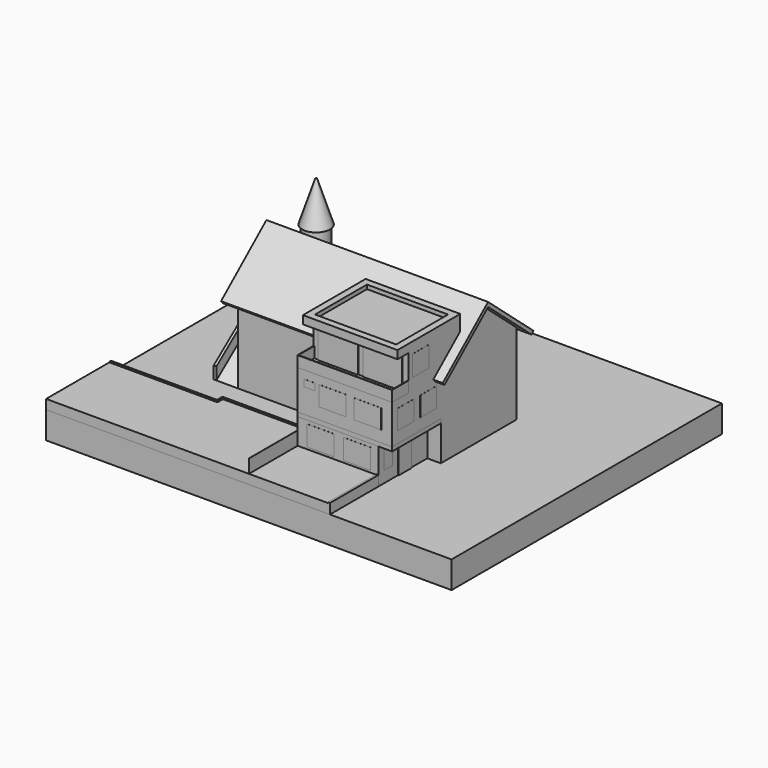
from build123d import *

# Parameters (mm, degrees)
F0_W      = 14000
F0_H      = 7000
F1_DEPTH  = 6000
F3_DEPTH  = 14000
F4_DEPTH  = 250
F5_DEPTH  = 250
F7_DEPTH  = 14000
F8_DEPTH  = 700
F9_DEPTH  = 700
F11_DEPTH = 700
F13_DEPTH = 700
F14_W     = 7000
F14_H     = 4500
F15_DEPTH = 9000
F16_DEPTH = 1800
F17_W     = 7000
F17_H     = 2600
F18_DEPTH = 1500
F19_DEPTH = 500
F20_W     = 6000
F20_H     = 4800
F21_DEPTH = 300
F22_W     = 7000
F22_H     = 300
F23_DEPTH = 4500
F24_DEPTH = 4500
F26_DEPTH = 800
F27_W     = 4500
F27_H     = 2600.45170784
F28_DEPTH = 1000
F29_W     = 1200
F29_H     = 2100
F30_DEPTH = 50
F31_W     = 6235.3289425373
F31_H     = 2381.1943054199
F32_DEPTH = 50
F33_W     = 400
F33_H     = 2600
F34_DEPTH = 500
F35_W     = 1500
F35_H     = 500
F36_DEPTH = 5
F37_W     = 2000
F37_H     = 1500
F38_DEPTH = 5
F39_W     = 1500
F39_H     = 500
F40_DEPTH = 5
F41_W     = 800
F41_H     = 1450.45170784
F42_DEPTH = 5
F43_W     = 800
F43_H     = 500
F44_DEPTH = 5
F43_W_2   = 2000
F43_H_2   = 1450
F43_H_3   = 1420.1555252075
F45_W     = 1500
F45_H     = 1450
F46_DEPTH = 5
F47_W     = 1500
F47_H     = 1530
F48_DEPTH = 5
F49_W     = 2200
F49_H     = 500
F50_DEPTH = 5
F51_W     = 30000
F51_H     = 25000
F52_DEPTH = 2000
F53_W     = 150
F53_H     = 0.9212493896
F53_H_2   = 4500
F54_DEPTH = 750
F53_W_2   = 7000
F53_H_3   = 150
F53_H_4   = 4500.9212493896
F55_DEPTH = 700
F56_W     = 10
F56_H     = 4500.9212493896
F57_DEPTH = 1000
F58_DEPTH = 1000
F59_DEPTH = 1000
F61_DEPTH = 1800
F63_DEPTH = 2000
F64_DEPTH = 50
F65_DEPTH = 50
F67_DEPTH = 2000
F68_DEPTH = 100
F69_DEPTH = 100
F71_DEPTH = 6000
F73_DEPTH = 200
F74_R     = 900
F75_DEPTH = 8500
F76_R     = 1050
F77_DEPTH = 3000


# Not quite as in the source:
# - a fillet or chamfer that OpenCascade refuses, or shapes differently, is made with other operations: its cross-section is extruded or revolved along the edge and cut away or added


with BuildPart() as f1:
    # F0 (on Top) → F1 (new body)
    with BuildSketch(Plane.XY):
        Rectangle(F0_W, F0_H)
    extrude(amount=F1_DEPTH)

    # F2 (on face) → F3 (join)
    with BuildSketch(Plane(origin=(-7000, 0, 0), x_dir=(0, -1, 0), z_dir=(-1, 0, 0))):
        Polygon((-3500, 6000), (0, 6000), (0, 8988.2593154907), align=None)
        Polygon((0, 8988.2593154907), (0, 6000), (3500, 6000), align=None)
    extrude(amount=-F3_DEPTH)

    # F4 (add, symmetric): a face of the model
    f4_faces = [f1.faces().sort_by_distance(p)[0] for p in [
        (0, 1750, 7494.1296577454),
    ]]
    extrude(f4_faces, amount=F4_DEPTH, both=True)

    # F5 (add, symmetric): a face of the model
    f5_faces = [f1.faces().sort_by_distance(p)[0] for p in [
        (0, -1750, 7494.1296577454),
    ]]
    extrude(f5_faces, amount=F5_DEPTH, both=True)

    # F6 (on face) → F7 (join)
    with BuildSketch(Plane(origin=(-7000, 0, 0), x_dir=(0, -1, 0), z_dir=(-1, 0, 0))):
        Polygon((0, 9316.9836101839), (-162.3298744643, 9178.3882503123), (0, 8988.2593154907), (162.3298744643, 9178.3882503123), align=None)
    extrude(amount=-F7_DEPTH)

    # F8 (add): a face of the model
    f8_faces = [f1.faces().sort_by_distance(p)[0] for p in [
        (0, 3581.1649372321, 6095.0644674108),
    ]]
    extrude(f8_faces, amount=F8_DEPTH)

    # F9 (add): a face of the model
    f9_faces = [f1.faces().sort_by_distance(p)[0] for p in [
        (0, -3581.1649372321, 6095.0644674108),
    ]]
    extrude(f9_faces, amount=F9_DEPTH)

    # F10 (on face) → F11 (join)
    with BuildSketch(Plane(origin=(-7000, 0, 0), x_dir=(0, -1, 0), z_dir=(-1, 0, 0))):
        Polygon((-4032.3610175005, 5545.4763515), (-3500, 6000), (0, 8917.555809021), (3500, 6000), (4032.3610175005, 5545.4763515), (4194.6908919648, 5735.6052863216), (0, 9316.9836101839), (-4194.6908919648, 5735.6052863216), align=None)
    extrude(amount=F11_DEPTH)

    # F12 (on face) → F13 (join)
    with BuildSketch(Plane.YZ.offset(7000)):
        Polygon((-4032.3610175005, 5545.4763515), (-3500, 6000), (0, 8988.2593154907), (3500, 6000), (4032.3610175005, 5545.4763515), (4194.6908919648, 5735.6052863216), (0, 9316.9836101839), (-4194.6908919648, 5735.6052863216), align=None)
    extrude(amount=F13_DEPTH)

    # F14 (on face) → F15 (join)
    with BuildSketch(Plane(origin=(0, 0, 0), x_dir=(1, 0, 0), z_dir=(0, 0, -1))):
        with Locations((3500, 5750)):
            Rectangle(F14_W, F14_H)
    extrude(amount=-F15_DEPTH)

    # F16 (add): a face of the model
    f16_faces = [f1.faces().sort_by_distance(p)[0] for p in [
        (3500, -3500, 7664.3621473466),
    ]]
    extrude(f16_faces, amount=F16_DEPTH)

    # F17 (on face) → F18 (cut)
    with BuildSketch(Plane.XZ.offset(8000)):
        with Locations((3500, 7100)):
            Rectangle(F17_W, F17_H)
    extrude(amount=-F18_DEPTH, mode=Mode.SUBTRACT)

    # F19 (cut): a face of the model
    f19_faces = [f1.faces().sort_by_distance(p)[0] for p in [
        (3500, -8000, 8700),
    ]]
    extrude(f19_faces, amount=-F19_DEPTH, mode=Mode.SUBTRACT)

    # F20 (on face) → F21 (cut)
    with BuildSketch(Plane.XY.offset(9000)):
        with Locations((3500, -4600)):
            Rectangle(F20_W, F20_H)
    extrude(amount=-F21_DEPTH, mode=Mode.SUBTRACT)


with BuildPart() as f23:
    # F22 (on face) → F23 (new body)
    with BuildSketch(Plane.XZ.offset(8000)):
        with Locations((3500, 2750)):
            Rectangle(F22_W, F22_H)
    extrude(amount=-F23_DEPTH)


with BuildPart() as f24:
    # F22 (on face) → F24 (new body)
    with BuildSketch(Plane.XZ.offset(8000)):
        with Locations((3500, 5650)):
            Rectangle(F22_W, F22_H)
    extrude(amount=-F24_DEPTH)


with BuildPart() as f26:
    # F25 (on face) → F26 (new body)
    with BuildSketch(Plane.XY.offset(5800)):
        Polygon((6960, -7960), (40, -7960), (40, -6500), (0, -6500), (0, -8000), (7000, -8000), (7000, -6500), (6960, -6500), align=None)
    extrude(amount=F26_DEPTH)


with BuildPart() as f28_tool:
    # F27 (on face) → F28 (new body)
    with BuildSketch(Plane.YZ.offset(7000)):
        with Locations((-5750, 1300.22585392)):
            Rectangle(F27_W, F27_H)
    extrude(amount=-F28_DEPTH)


with BuildPart() as f1_1:
    add(f1.part)

    # F28: cut by f28_tool
    add(f28_tool.part, mode=Mode.SUBTRACT)

    # F51 (on face) → F52 (join)
    with BuildSketch(Plane(origin=(0, 0, 0), x_dir=(1, 0, 0), z_dir=(0, 0, -1))):
        Rectangle(F51_W, F51_H)
    extrude(amount=F52_DEPTH)

    # F58 (add): a face of the model
    f58_faces = [f1_1.faces().sort_by_distance(p)[0] for p in [
        (-7000, 0, 3776.9399273598),
    ]]
    extrude(f58_faces, amount=F58_DEPTH)

    # F59 (add): a face of the model
    f59_faces = [f1_1.faces().sort_by_distance(p)[0] for p in [
        (-7700, 4043.5725637348, 5700.2662109964),
    ]]
    extrude(f59_faces, amount=F59_DEPTH)

    # F60 (on face) → F61 (join)
    with BuildSketch(Plane(origin=(-8000, 0, 0), x_dir=(0, -1, 0), z_dir=(-1, 0, 0))):
        Polygon((-2000, 0), (3500, 0), (1224.4793365597, 1777.8315871649), (1224.4793365597, 4500), (-2000, 4500), align=None)
    extrude(amount=F61_DEPTH)

    # F62 (on face) → F63 (join)
    with BuildSketch(Plane(origin=(-8000, 0, 0), x_dir=(0, -1, 0), z_dir=(-1, 0, 0))):
        Polygon((1224.4793365597, 4500), (-387.7603317201, 5825.6425857544), (-2000, 4500), align=None)
    extrude(amount=F63_DEPTH)

    # F64 (add): a face of the model
    f64_faces = [f1_1.faces().sort_by_distance(p)[0] for p in [
        (-9000, -418.3595024198, 5162.8212928772),
    ]]
    extrude(f64_faces, amount=F64_DEPTH)

    # F65 (add): a face of the model
    f65_faces = [f1_1.faces().sort_by_distance(p)[0] for p in [
        (-9000, 1193.8801658601, 5162.8212928772),
    ]]
    extrude(f65_faces, amount=F65_DEPTH)

    # F66 (on face) → F67 (join)
    with BuildSketch(Plane(origin=(-10000, 0, 0), x_dir=(0, -1, 0), z_dir=(-1, 0, 0))):
        Polygon((-387.7603317201, 5890.3742076897), (-419.5159347551, 5864.263586206), (-387.7603317201, 5825.6425857544), (-356.0047286852, 5864.263586206), align=None)
    extrude(amount=-F67_DEPTH)

    # F68 (add): a face of the model
    f68_faces = [f1_1.faces().sort_by_distance(p)[0] for p in [
        (-9000, 2015.8778015175, 4519.3105002258),
    ]]
    extrude(f68_faces, amount=F68_DEPTH)

    # F69 (add): a face of the model
    f69_faces = [f1_1.faces().sort_by_distance(p)[0] for p in [
        (-9000, -1240.3571380772, 4519.3105002258),
    ]]
    extrude(f69_faces, amount=F69_DEPTH)

    # F70 (on face) → F71 (cut)
    with BuildSketch(Plane.XZ.offset(3500)):
        Polygon((-10200, 4190.3742076897), (-8400, 5990.3742076897), (-10200, 5990.3742076897), align=None)
    extrude(amount=-F71_DEPTH, mode=Mode.SUBTRACT)

    # F72 (on face) → F73 (join)
    with BuildSketch(Plane(origin=(-9800, 0, 0), x_dir=(0, -1, 0), z_dir=(-1, 0, 0))):
        Polygon((1224.4793365597, 2685.697555542), (1224.4793365597, 1777.8315871649), (3500, 0), (3500, 907.8659683771), align=None)
    extrude(amount=-F73_DEPTH)

    # F74 (on face) → F75 (join)
    with BuildSketch(Plane.XY):
        with Locations((-7100, 2600)):
            Circle(F74_R)
    extrude(amount=F75_DEPTH)

    # F76 (on face) → F77 (join)
    with BuildSketch(Plane.XY.offset(8500)):
        with Locations((-7100, 2600)):
            Circle(F76_R)
    extrude(amount=F77_DEPTH)

    # F78: chamfer of 1000 x 3077.6835371753 on 1 edges, made by hand

    # F78_s1 → F78_t2 (revolve, cut)
    with BuildSketch(Plane.XZ.offset(-2600)):
        Polygon((-6050, 8422.3164628247), (-7050, 11500), (-6050, 11500), align=None)
    revolve(axis=Axis((-7100, 2600, 11500), (0, 0, 1)), mode=Mode.SUBTRACT)


with BuildPart() as f23_1:
    add(f23.part)

    # F28: cut by f28_tool
    add(f28_tool.part, mode=Mode.SUBTRACT)


with BuildPart() as f30:
    # F29 (on face) → F30 (new body, symmetric)
    with BuildSketch(Plane.YZ.offset(6000)):
        with Locations((-5600, 1050)):
            Rectangle(F29_W, F29_H)
    extrude(amount=F30_DEPTH, both=True)


with BuildPart() as f32:
    # F31 (on face) → F32 (new body, symmetric)
    with BuildSketch(Plane.XZ.offset(6500)):
        with Locations((3466.3508981466, 6990.59715271)):
            Rectangle(F31_W, F31_H)
    extrude(amount=F32_DEPTH, both=True)

    # F33 (on face) → F34 (cut)
    with BuildSketch(Plane.XZ.offset(6500)):
        with Locations((3500, 7100)):
            Rectangle(F33_W, F33_H)
    extrude(amount=F34_DEPTH, mode=Mode.SUBTRACT)


with BuildPart() as f36:
    # F35 (on face) → F36 (new body, symmetric)
    with BuildSketch(Plane(origin=(0, 0, 0), x_dir=(0, -1, 0), z_dir=(-1, 0, 0))):
        with Locations((6750, 2150)):
            Rectangle(F35_W, F35_H)
    extrude(amount=F36_DEPTH, both=True)


with BuildPart() as f36b:
    # F35 (on face) → F36, piece 2 (new body, symmetric)
    with BuildSketch(Plane(origin=(0, 0, 0), x_dir=(0, -1, 0), z_dir=(-1, 0, 0))):
        with Locations((4750, 2150)):
            Rectangle(F35_W, F35_H)
    extrude(amount=F36_DEPTH, both=True)


with BuildPart() as f38:
    # F37 (on face) → F38 (new body, symmetric)
    with BuildSketch(Plane.XZ.offset(8000)):
        with Locations((1700, 1600)):
            Rectangle(F37_W, F37_H)
    extrude(amount=F38_DEPTH, both=True)


with BuildPart() as f38b:
    # F37 (on face) → F38, piece 2 (new body, symmetric)
    with BuildSketch(Plane.XZ.offset(8000)):
        with Locations((4400, 1600)):
            Rectangle(F37_W, F37_H)
    extrude(amount=F38_DEPTH, both=True)


with BuildPart() as f40:
    # F39 (on face) → F40 (new body, symmetric)
    with BuildSketch(Plane(origin=(0, 0, 0), x_dir=(0, -1, 0), z_dir=(-1, 0, 0))):
        with Locations((4750, 4950)):
            Rectangle(F39_W, F39_H)
    extrude(amount=F40_DEPTH, both=True)


with BuildPart() as f40b:
    # F39 (on face) → F40, piece 2 (new body, symmetric)
    with BuildSketch(Plane(origin=(0, 0, 0), x_dir=(0, -1, 0), z_dir=(-1, 0, 0))):
        with Locations((6750, 4950)):
            Rectangle(F39_W, F39_H)
    extrude(amount=F40_DEPTH, both=True)


with BuildPart() as f42:
    # F41 (on face) → F42 (new body, symmetric)
    with BuildSketch(Plane.YZ.offset(6000)):
        with Locations((-7100, 1575.22585392)):
            Rectangle(F41_W, F41_H)
    extrude(amount=F42_DEPTH, both=True)


with BuildPart() as f44:
    # F43 (on face) → F44 (new body, symmetric)
    with BuildSketch(Plane.XZ.offset(8000)):
        with Locations((900, 4950)):
            Rectangle(F43_W, F43_H)
    extrude(amount=F44_DEPTH, both=True)


with BuildPart() as f44b:
    # F43 (on face) → F44, piece 2 (new body, symmetric)
    with BuildSketch(Plane.XZ.offset(8000)):
        with Locations((2600, 4475)):
            Rectangle(F43_W_2, F43_H_2)
    extrude(amount=F44_DEPTH, both=True)


with BuildPart() as f44c:
    # F43 (on face) → F44, piece 3 (new body, symmetric)
    with BuildSketch(Plane.XZ.offset(8000)):
        with Locations((5200, 4460.0777626038)):
            Rectangle(F43_W_2, F43_H_3)
    extrude(amount=F44_DEPTH, both=True)


with BuildPart() as f46:
    # F45 (on face) → F46 (new body, symmetric)
    with BuildSketch(Plane.YZ.offset(7000)):
        with Locations((-6750, 4475)):
            Rectangle(F45_W, F45_H)
    extrude(amount=F46_DEPTH, both=True)


with BuildPart() as f46b:
    # F45 (on face) → F46, piece 2 (new body, symmetric)
    with BuildSketch(Plane.YZ.offset(7000)):
        with Locations((-4650, 4475)):
            Rectangle(F45_W, F45_H)
    extrude(amount=F46_DEPTH, both=True)


with BuildPart() as f48:
    # F47 (on face) → F48 (new body, symmetric)
    with BuildSketch(Plane.YZ.offset(7000)):
        with Locations((-5350, 7415)):
            Rectangle(F47_W, F47_H)
    extrude(amount=F48_DEPTH, both=True)


with BuildPart() as f50:
    # F49 (on face) → F50 (new body, symmetric)
    with BuildSketch(Plane(origin=(0, 0, 0), x_dir=(0, -1, 0), z_dir=(-1, 0, 0))):
        with Locations((5000, 7931.1943054199)):
            Rectangle(F49_W, F49_H)
    extrude(amount=F50_DEPTH, both=True)


with BuildPart() as f54:
    # F53 (on face) → F54 (new body)
    with BuildSketch(Plane.XY):
        with Locations((5925, -7999.5393753052)):
            Rectangle(F53_W, F53_H)
        with Locations((5925, -10250)):
            Rectangle(F53_W, F53_H_2)
    extrude(amount=F54_DEPTH)


with BuildPart() as f54b:
    # F53 (on face) → F54, piece 2 (new body)
    with BuildSketch(Plane.XY):
        with Locations((-3500, -6075)):
            Rectangle(F53_W_2, F53_H_3)
        Polygon((-7000, -6150), (-7000, -6000), (-7150, -6000), (-7150, -6500), (-15000, -6500), (-15000, -6650), (-7000, -6650), align=None)
    extrude(amount=F54_DEPTH)


with BuildPart() as f55:
    # F53 (on face) → F55 (new body)
    with BuildSketch(Plane.XY):
        with Locations((-3500, -6075)):
            Rectangle(F53_W_2, F53_H_3)
        Polygon((-7000, -6150), (-7000, -6000), (-7150, -6000), (-7150, -6500), (-15000, -6500), (-15000, -6650), (-7000, -6650), align=None)
        Polygon((0, -7999.0787506104), (0, -6150), (-7000, -6150), (-7000, -6650), (-15000, -6650), (-15000, -12500), (5850, -12500), (5850, -7999.0787506104), align=None)
        with Locations((5925, -10249.5393753052)):
            Rectangle(F53_W, F53_H_4)
    extrude(amount=F55_DEPTH)


with BuildPart() as f57:
    # F56 (on face) → F57 (new body)
    with BuildSketch(Plane.XY.offset(700)):
        with Locations((5, -10249.5393753052)):
            Rectangle(F56_W, F56_H)
    extrude(amount=F57_DEPTH)


solid = Compound([f24.part, f26.part, f1_1.part, f23_1.part, f30.part, f32.part, f36.part, f36b.part, f38.part, f38b.part, f40.part, f40b.part, f42.part, f44.part, f44b.part, f44c.part, f46.part, f46b.part, f48.part, f50.part, f54.part, f54b.part, f55.part, f57.part])
